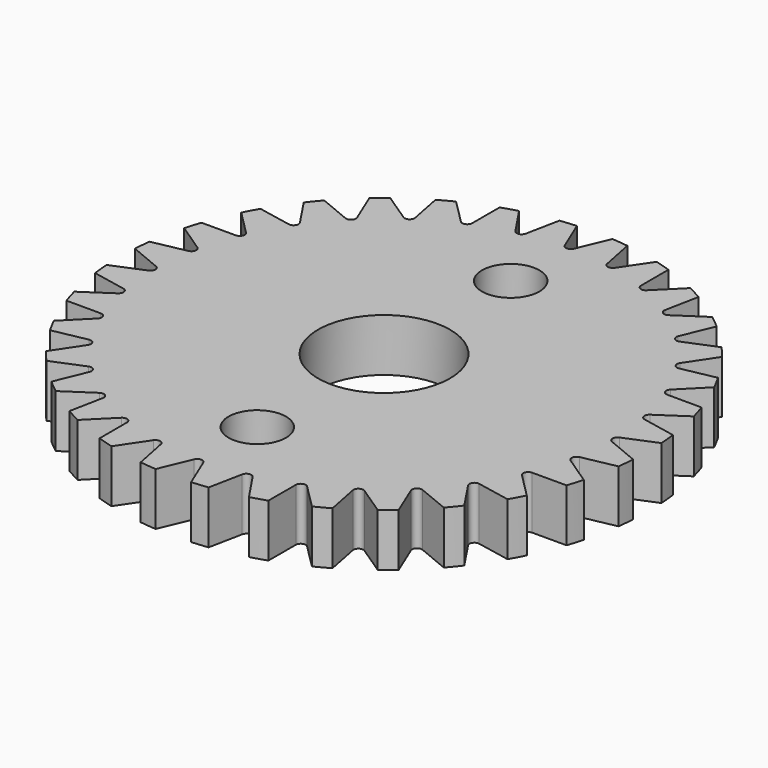
from build123d import *

# Parameters (mm, degrees)
F0_R            = 15.8688012495
F0_R_2          = 1.7272
F0_R_3          = 3.96875
F1_DEPTH        = 3.175
F3_DEPTH        = 3.175
F3_COPIES_COUNT = 32


# Not quite as in the source:
# - a pattern or mirror of a feature is missing from the dataset's text; its kind, count and spacing are read off the source's solid


with BuildPart() as f1:
    # F0 (on Top) → F1 (new body)
    with BuildSketch(Plane.XY):
        Circle(F0_R)
        with Locations((0, -9.525)):
            Circle(F0_R_2, mode=Mode.SUBTRACT)
        Circle(F0_R_3, mode=Mode.SUBTRACT)
        with Locations((0, 9.525)):
            Circle(F0_R_2, mode=Mode.SUBTRACT)
    extrude(amount=F1_DEPTH)

    # F2 (on face) → F3 (cut, through all)
    with BuildSketch(Plane.XY.offset(3.175)):
        with BuildLine():
            Line((-13.9312413972, 0.274735453), (-15.8329891451, 1.065508248))
            ThreePointArc((-15.8329891451, 1.065508248), (-15.8688012495, 0), (-15.8329891451, -1.065508248))
            Line((-15.8329891451, -1.065508248), (-13.9312413972, -0.274735453))
            ThreePointArc((-13.9312413972, -0.274735453), (-13.747940143, 0), (-13.9312413972, 0.274735453))
        make_face()
    f3 = extrude(amount=-F3_DEPTH, mode=Mode.SUBTRACT)

    # F3_copies: F3 ×32 about axis
    f3_copies_axis = Axis((0, 0, 0), (0, 0, 1))
    for i in range(1, F3_COPIES_COUNT):
        add(f3.rotate(f3_copies_axis, i * 360 / F3_COPIES_COUNT), mode=Mode.SUBTRACT)


solid = f1.part
